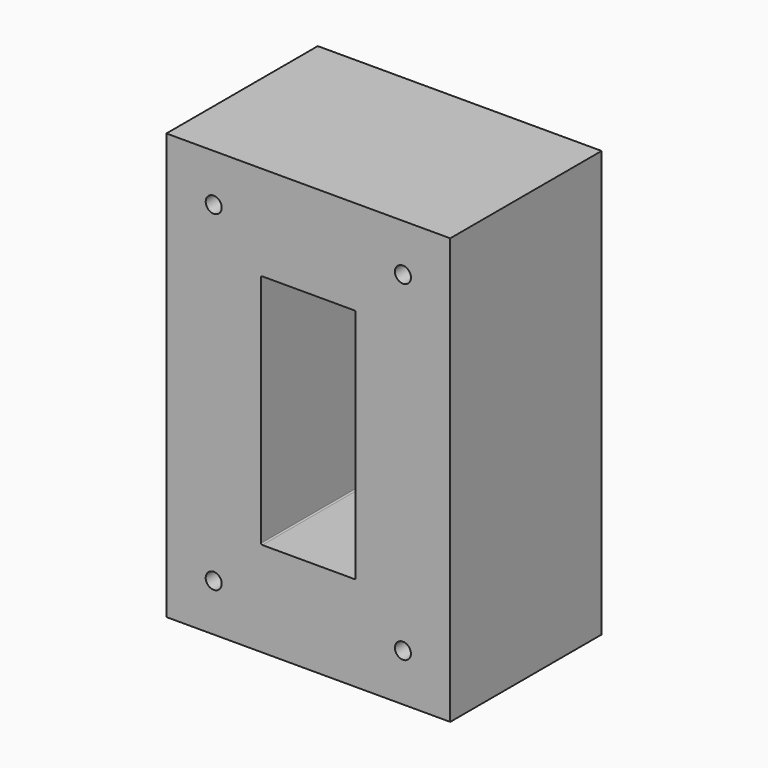
from build123d import *

# Parameters (mm, degrees)
F1_W     = 182.88
F1_H     = 274.32
F2_DEPTH = 121.92
F3_R     = 5.159375
F4_DEPTH = 121.92
F5_W     = 60.96
F5_H     = 152.4
F6_DEPTH = 121.92
F7_R     = 0.79375


with BuildPart() as f2:
    # F1 (on Front) → F2 (new body)
    with BuildSketch(Plane.XZ):
        Rectangle(F1_W, F1_H)
    extrude(amount=-F2_DEPTH)

    # F3 (on face) → F4 (cut)
    with BuildSketch(Plane.XZ):
        with Locations((-60.96, 106.68)):
            Circle(F3_R)
        with Locations((60.96, 106.68)):
            Circle(F3_R)
        with Locations((-60.96, -106.68)):
            Circle(F3_R)
        with Locations((60.96, -106.68)):
            Circle(F3_R)
    extrude(amount=-F4_DEPTH, mode=Mode.SUBTRACT)

    # F5 (on face) → F6 (cut)
    with BuildSketch(Plane.XZ):
        Rectangle(F5_W, F5_H)
    extrude(amount=-F6_DEPTH, mode=Mode.SUBTRACT)

    # F7
    f7_edges = [f2.edges().sort_by_distance(p)[0] for p in [
        (-30.48, 60.96, 76.2),
        (30.48, 60.96, 76.2),
        (30.48, 60.96, -76.2),
        (-30.48, 60.96, -76.2),
    ]]
    fillet(f7_edges, radius=F7_R)


solid = f2.part
